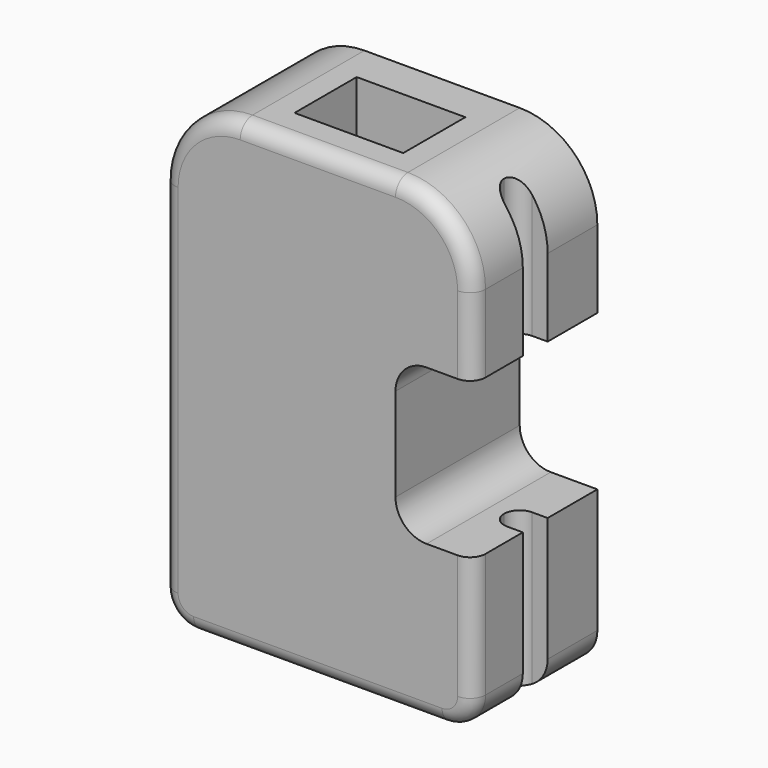
from build123d import *

# Parameters (mm, degrees)
F1_DEPTH  = 10
F2_R      = 1
F3_W      = 2
F3_H      = 2
F4_DEPTH  = 20
F5_R      = 2
F6_R      = 2
F7_W      = 7
F7_H      = 5
F8_DEPTH  = 8
F9_R      = 0.99999
F10_W     = 9
F10_H     = 4
F11_DEPTH = 6


# Not quite as in the source:
# - a fillet or chamfer is up to 0.001 mm smaller than in the source, because OpenCascade refuses the exact size


with BuildPart() as f1:
    # F0 (on Front) → F1 (new body)
    with BuildSketch(Plane.XZ):
        with BuildLine():
            Line((-18, 0), (-2, 0))
            ThreePointArc((-2, 0), (-0.5857864376, 0.5857864376), (0, 2))
            Line((0, 2), (0, 10))
            Line((0, 10), (-5, 10))
            Line((-5, 10), (-5, 20))
            Line((-5, 20), (0, 20))
            Line((0, 20), (0, 25))
            ThreePointArc((0, 25), (-1.4644660941, 28.5355339059), (-5, 30))
            Line((-5, 30), (-15, 30))
            ThreePointArc((-15, 30), (-18.5355339059, 28.5355339059), (-20, 25))
            Line((-20, 25), (-20, 2))
            ThreePointArc((-20, 2), (-19.4142135624, 0.5857864376), (-18, 0))
        make_face()
    extrude(amount=F1_DEPTH)

    # F2
    f2_edges = [f1.edges().sort_by_distance(p)[0] for p in [
        (-10, -10, 30),
    ]]
    fillet(f2_edges, radius=F2_R)

    # F3 (on face) → F4 (cut, symmetric)
    with BuildSketch(Plane(origin=(0, 0, 20), x_dir=(1, 0, 0), z_dir=(0, 0, -1))):
        with Locations((-1, 5)):
            Rectangle(F3_W, F3_H)
    extrude(amount=F4_DEPTH, both=True, mode=Mode.SUBTRACT)

    # F5
    f5_edges = [f1.edges().sort_by_distance(p)[0] for p in [
        (-5, -5, 20),
    ]]
    fillet(f5_edges, radius=F5_R)

    # F6
    f6_edges = [f1.edges().sort_by_distance(p)[0] for p in [
        (-5, -5, 10),
    ]]
    fillet(f6_edges, radius=F6_R)

    # F7 (on face) → F8 (cut)
    with BuildSketch(Plane.XY.offset(30)):
        with Locations((-10, -5)):
            Rectangle(F7_W, F7_H)
    extrude(amount=-F8_DEPTH, mode=Mode.SUBTRACT)

    # F9 (radius 1 in the source; OpenCascade refuses exactly that, so slightly less here)
    f9_edges = [f1.edges().sort_by_distance(p)[0] for p in [
        (-2, -4, 24.5),
        (-2, -6, 24.5),
        (-2, -6, 5),
        (-2, -4, 5),
    ]]
    fillet(f9_edges, radius=F9_R)

    # F10 (on face) → F11 (cut)
    with BuildSketch(Plane(origin=(0, 0, 0), x_dir=(1, 0, 0), z_dir=(0, 0, -1))):
        with Locations((-10, 5)):
            Rectangle(F10_W, F10_H)
    extrude(amount=-F11_DEPTH, mode=Mode.SUBTRACT)


solid = f1.part
